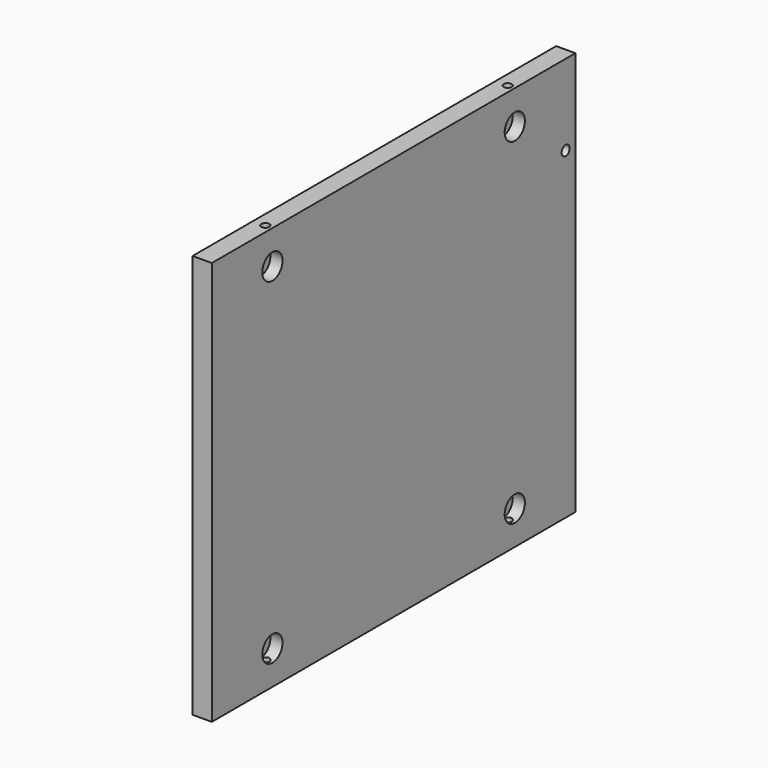
from build123d import *

# Parameters (mm, degrees)
F0_W     = 450
F0_H     = 400
F1_DEPTH = 19
F2_R     = 12.5
F3_DEPTH = 12
F5_D     = 8
F5_DEPTH = 22
F5_TIP   = 2.4034424761
F7_D     = 10
F7_DEPTH = 13
F7_TIP   = 3.0043030951


# Not quite as in the source:
# - a pattern or mirror of a feature is missing from the dataset's text; its kind, count and spacing are read off the source's solid


with BuildPart() as f1:
    # F0 (on Right) → F1 (new body)
    with BuildSketch(Plane.YZ):
        Rectangle(F0_W, F0_H)
    extrude(amount=-F1_DEPTH)

    # F2 (on face) → F3 (cut)
    with BuildSketch(Plane.YZ):
        with Locations((-150, -166.5)):
            Circle(F2_R)
        with Locations((150, -166.5)):
            Circle(F2_R)
        with Locations((-150, 166.5)):
            Circle(F2_R)
        with Locations((150, 166.5)):
            Circle(F2_R)
    extrude(amount=-F3_DEPTH, mode=Mode.SUBTRACT)

    # F5
    with Locations(Plane.XY.offset(200)):
        with Locations((-7, 150), (-7, -150)):
            f5 = Hole(F5_D / 2, depth=F5_DEPTH)
            with Locations((0, 0, -(F5_DEPTH + F5_TIP / 2))):  # 118° drill point
                Cone(0, F5_D / 2, F5_TIP, mode=Mode.SUBTRACT)

    # F5_copies: F5 across plane
    add(f5.mirror(Plane(origin=(0, 0, 2.1e-05), x_dir=(-1, 0, 0), z_dir=(0, 0, -1))), mode=Mode.SUBTRACT)

    # F7
    with Locations(Plane.YZ):
        with Locations((213, 120)):
            Hole(F7_D / 2, depth=F7_DEPTH)
            with Locations((0, 0, -(F7_DEPTH + F7_TIP / 2))):  # 118° drill point
                Cone(0, F7_D / 2, F7_TIP, mode=Mode.SUBTRACT)


solid = f1.part
